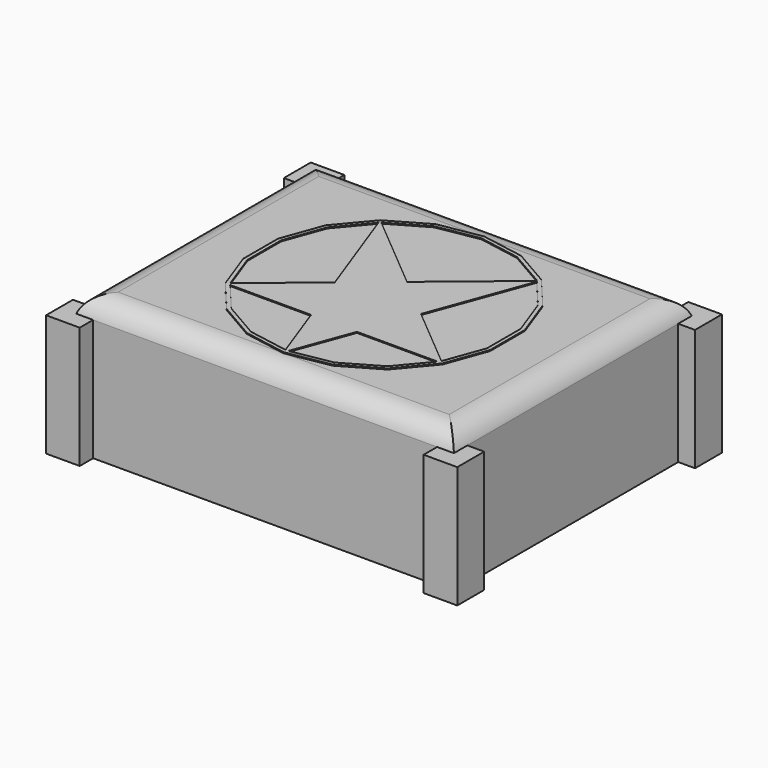
from build123d import *

# Parameters (mm, degrees)
F0_W        = 77.5
F0_H        = 61
F1_DEPTH    = 3.5
F2_T1_DEPTH = 84.8484800354
F2_T3_DEPTH = 101.3484800354
F5_DEPTH    = 25
F6_DEPTH    = 0.2


# Not quite as in the source:
# - a fillet or chamfer that OpenCascade refuses, or shapes differently, is made with other operations: its cross-section is extruded or revolved along the edge and cut away or added


with BuildPart() as f1:
    # F0 (on Top) → F1 (new body)
    with BuildSketch(Plane.XY):
        Rectangle(F0_W, F0_H)
    extrude(amount=F1_DEPTH)

    # F2: fillet of radius 5 on 4 edges, made by hand

    # F2_s2 → F2_t1 (cut)
    with BuildSketch(Plane.XZ.offset(-42.4242400177)):
        with BuildLine():
            ThreePointArc((38.75, 0), (36.9383438845, 2.5311288741), (33.9803039929, 3.5))
            Line((33.9803039929, 3.5), (38.75, 3.5))
            Line((38.75, 3.5), (38.75, 0))
        make_face()
        with BuildLine():
            ThreePointArc((-38.75, 0), (-36.9383438845, 2.5311288741), (-33.9803039929, 3.5))
            Line((-33.9803039929, 3.5), (-38.75, 3.5))
            Line((-38.75, 3.5), (-38.75, 0))
        make_face()
    extrude(amount=F2_T1_DEPTH, mode=Mode.SUBTRACT)

    # F2_s4 → F2_t3 (cut)
    with BuildSketch(Plane.YZ.offset(-50.6742400177)):
        with BuildLine():
            ThreePointArc((30.5, 0), (28.6883438845, 2.5311288741), (25.7303039929, 3.5))
            Line((25.7303039929, 3.5), (30.5, 3.5))
            Line((30.5, 3.5), (30.5, 0))
        make_face()
        with BuildLine():
            ThreePointArc((-30.5, 0), (-28.6883438845, 2.5311288741), (-25.7303039929, 3.5))
            Line((-25.7303039929, 3.5), (-30.5, 3.5))
            Line((-30.5, 3.5), (-30.5, 0))
        make_face()
    extrude(amount=F2_T3_DEPTH, mode=Mode.SUBTRACT)

    # F4 (on face) → F5 (join)
    with BuildSketch(Plane(origin=(0, 0, 0), x_dir=(1, 0, 0), z_dir=(0, 0, -1))):
        Polygon((-38.75, 29.5), (-38.75, 30.5), (-37.75, 30.5), (-35.3, 30.5), (-35.3, 33.95), (-42.2, 33.95), (-42.2, 27.05), (-38.75, 27.05), align=None)
        Polygon((-37.75, 30.5), (-38.75, 30.5), (-38.75, 29.5), (-38.75, 27.05), (-38.75, -27.05), (-38.75, -29.5), (-38.75, -30.5), (-37.75, -30.5), (-35.3, -30.5), (35.3, -30.5), (37.75, -30.5), (38.75, -30.5), (38.75, -29.5), (38.75, -27.05), (38.75, 27.05), (38.75, 29.5), (38.75, 30.5), (37.75, 30.5), (35.3, 30.5), (-35.3, 30.5), align=None)
        Polygon((-35.3, 27.05), (-35.3, 29.5), (35.3, 29.5), (35.3, 27.05), (37.75, 27.05), (37.75, -27.05), (35.3, -27.05), (35.3, -29.5), (-35.3, -29.5), (-35.3, -27.05), (-37.75, -27.05), (-37.75, 27.05), align=None, mode=Mode.SUBTRACT)
        Polygon((35.3, 33.95), (35.3, 30.5), (37.75, 30.5), (38.75, 30.5), (38.75, 29.5), (38.75, 27.05), (42.2, 27.05), (42.2, 33.95), align=None)
        Polygon((-38.75, -29.5), (-38.75, -27.05), (-42.2, -27.05), (-42.2, -33.95), (-35.3, -33.95), (-35.3, -30.5), (-37.75, -30.5), (-38.75, -30.5), align=None)
        Polygon((42.2, -27.05), (38.75, -27.05), (38.75, -29.5), (38.75, -30.5), (37.75, -30.5), (35.3, -30.5), (35.3, -33.95), (42.2, -33.95), align=None)
    extrude(amount=F5_DEPTH)

    # F3 (on face) → F6 (join)
    with BuildSketch(Plane.XY.offset(3.5)):
        Polygon((-16.2400073105, 18.8887493843), (-8.7504151188, -1.6887360431), (0.1768791019, 5.6841672089), (-15.9216975961, 19.1924769786), (-16.0447749761, 19.1214182202), align=None)
        Polygon((-21.294405657, -12.8651519965), (-4.682532386, -12.8651519965), (-8.7504151188, -1.6887360431), (-21.6633903185, -12.3533466729), (-21.6170668475, -12.4806193635), align=None)
        Polygon((-4.682532386, -12.8651519965), (-0.2991132897, -24.9084969837), (0, -24.961238727), (0.3027663667, -24.9078528477), (4.7360081498, -12.8651519965), align=None)
        Polygon((8.8770657691, -1.6161562148), (4.7360081498, -12.8651519965), (21.294405657, -12.8651519965), (21.6170668475, -12.4806193635), (21.665673901, -12.3470725815), align=None)
        Polygon((0.1768791019, 5.6841672089), (8.8770657691, -1.6161562148), (16.3689174848, 18.7351202209), (16.20943331, 18.9251860592), align=None)
        Polygon((-25.3394028596, -4.4680203992), (-22.283096905, -12.8651519965), (-21.6633903185, -12.3533466729), (-24.5820214231, -4.3344736172), (-24.5820214231, 4.3344736172), (-21.6170668475, 12.4806193635), (-16.2400073105, 18.8887493843), (-16.5391206001, 19.7105563935), (-22.283096905, 12.8651519965), (-25.3394028596, 4.4680203992), align=None)
        Polygon((0.3027663667, -24.9078528477), (0, -25.7303039929), (8.8002822595, -24.1785767927), (16.5391206001, -19.7105563935), (22.283096905, -12.8651519965), (21.294405657, -12.8651519965), (16.0447749761, -19.1214182202), (8.537246447, -23.4558918374), align=None)
        Polygon((-8.8002822595, -24.1785767927), (0, -25.7303039929), (-0.2991132897, -24.9084969837), (-8.537246447, -23.4558918374), (-16.0447749761, -19.1214182202), (-21.294405657, -12.8651519965), (-22.283096905, -12.8651519965), (-16.5391206001, -19.7105563935), align=None)
        Polygon((-22.283096905, -12.8651519965), (-21.294405657, -12.8651519965), (-21.6170668475, -12.4806193635), (-21.6633903185, -12.3533466729), align=None)
        Polygon((-16.5391206001, 19.7105563935), (-16.2400073105, 18.8887493843), (-16.0447749761, 19.1214182202), (-15.9216975961, 19.1924769786), align=None)
        Polygon((21.665673901, -12.3470725815), (22.283096905, -12.8651519965), (25.3394028596, -4.4680203992), (25.3394028596, 4.4680203992), (22.283096905, 12.8651519965), (16.5391206001, 19.7105563935), (8.8002822595, 24.1785767927), (0, 25.7303039929), (-8.8002822595, 24.1785767927), (-16.5391206001, 19.7105563935), (-15.9216975961, 19.1924769786), (-8.537246447, 23.4558918374), (0, 24.961238727), (8.537246447, 23.4558918374), (16.0447749761, 19.1214182202), (16.20943331, 18.9251860592), (16.5391206001, 19.1974692878), (16.3689174848, 18.7351202209), (21.6170668475, 12.4806193635), (24.5820214231, 4.3344736172), (24.5820214231, -4.3344736172), align=None)
        Polygon((16.20943331, 18.9251860592), (16.3689174848, 18.7351202209), (16.5391206001, 19.1974692878), align=None)
        Polygon((21.6170668475, -12.4806193635), (21.294405657, -12.8651519965), (22.283096905, -12.8651519965), (21.665673901, -12.3470725815), align=None)
        Polygon((-0.2991132897, -24.9084969837), (0, -25.7303039929), (0.3027663667, -24.9078528477), (0, -24.961238727), align=None)
        Polygon((-8.7504151188, -1.6887360431), (-4.682532386, -12.8651519965), (4.7360081498, -12.8651519965), (8.8770657691, -1.6161562148), (0.1768791019, 5.6841672089), align=None)
    extrude(amount=F6_DEPTH)


solid = f1.part
